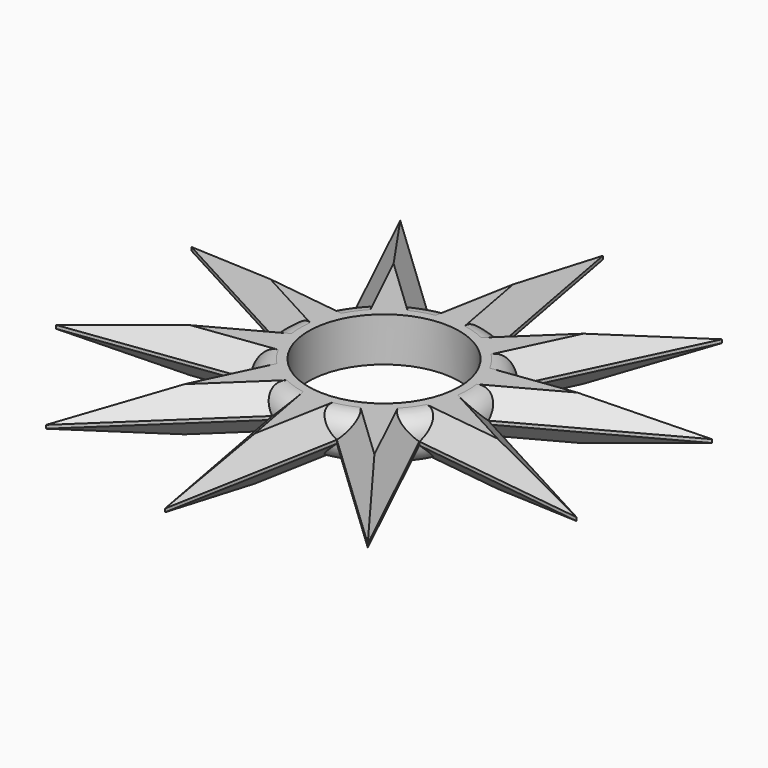
from build123d import *

# Parameters (mm, degrees)
F0_R     = 11.1
F1_DEPTH = 6.5
F2_SIZE  = 3
F3_R     = 2.99999


# Not quite as in the source:
# - a fillet or chamfer is up to 0.001 mm smaller than in the source, because OpenCascade refuses the exact size


with BuildPart() as f1:
    # F0 (on Top) → F1 (new body)
    with BuildSketch(Plane.XY):
        with BuildLine():
            Line((0, 40.2588956058), (-4.7404649607, 14.6152020464))
            ThreePointArc((-4.7404649607, 14.6152020464), (-4.7479748611, 14.612764065), (-4.7554835077, 14.6103222247))
            Line((-4.7554835077, 14.6103222247), (-23.6635851107, 32.5701307199))
            Line((-23.6635851107, 32.5701307199), (-12.4257169366, 9.0375714388))
            ThreePointArc((-12.4257169366, 9.0375714388), (-12.4303595641, 9.0311848617), (-12.4349989091, 9.0247958997))
            Line((-12.4349989091, 9.0247958997), (-38.2884850047, 12.440682917))
            Line((-38.2884850047, 12.440682917), (-15.3647673773, 0.0078957174))
            ThreePointArc((-15.3647673773, 0.0078957174), (-15.364769406, 0), (-15.3647673773, -0.0078957174))
            Line((-15.3647673773, -0.0078957174), (-38.2884850047, -12.440682917))
            Line((-38.2884850047, -12.440682917), (-12.4349989091, -9.0247958997))
            ThreePointArc((-12.4349989091, -9.0247958997), (-12.4303595641, -9.0311848617), (-12.4257169366, -9.0375714388))
            Line((-12.4257169366, -9.0375714388), (-23.6635851107, -32.5701307199))
            Line((-23.6635851107, -32.5701307199), (-4.7554835077, -14.6103222247))
            ThreePointArc((-4.7554835077, -14.6103222247), (-4.7479748611, -14.612764065), (-4.7404649607, -14.6152020464))
            Line((-4.7404649607, -14.6152020464), (0, -40.2588956058))
            Line((0, -40.2588956058), (4.7404649607, -14.6152020464))
            ThreePointArc((4.7404649607, -14.6152020464), (4.7479748611, -14.612764065), (4.7554835077, -14.6103222247))
            Line((4.7554835077, -14.6103222247), (23.6635851107, -32.5701307199))
            Line((23.6635851107, -32.5701307199), (12.4257169366, -9.0375714388))
            ThreePointArc((12.4257169366, -9.0375714388), (12.4303595641, -9.0311848617), (12.4349989091, -9.0247958997))
            Line((12.4349989091, -9.0247958997), (38.2884850047, -12.440682917))
            Line((38.2884850047, -12.440682917), (15.3647673773, -0.0078957174))
            ThreePointArc((15.3647673773, -0.0078957174), (15.364769406, 0), (15.3647673773, 0.0078957174))
            Line((15.3647673773, 0.0078957174), (38.2884850047, 12.440682917))
            Line((38.2884850047, 12.440682917), (12.4349989091, 9.0247958997))
            ThreePointArc((12.4349989091, 9.0247958997), (12.4303595641, 9.0311848617), (12.4257169366, 9.0375714388))
            Line((12.4257169366, 9.0375714388), (23.6635851107, 32.5701307199))
            Line((23.6635851107, 32.5701307199), (4.7554835077, 14.6103222247))
            ThreePointArc((4.7554835077, 14.6103222247), (4.7479748611, 14.612764065), (4.7404649607, 14.6152020464))
            Line((4.7404649607, 14.6152020464), (0, 40.2588956058))
        make_face()
        Circle(F0_R, mode=Mode.SUBTRACT)
    extrude(amount=F1_DEPTH)

    # F2
    f2_edges = [f1.edges().sort_by_distance(p)[0] for p in [
        (-26.826626, -6.224289, 6.5),
        (-26.826626, 6.224289, 6.5),
        (-25.361742, 10.732739, 6.5),
        (-18.044651, 20.803851, 6.5),
        (-14.209534, 23.590226, 6.5),
        (-2.370232, 27.437049, 6.5),
        (2.370232, 27.437049, 6.5),
        (14.209534, 23.590226, 6.5),
        (18.044651, 20.803851, 6.5),
        (25.361742, 10.732739, 6.5),
        (26.826626, 6.224289, 6.5),
        (26.826626, -6.224289, 6.5),
        (25.361742, -10.732739, 6.5),
        (18.044651, -20.803851, 6.5),
        (14.209534, -23.590226, 6.5),
        (2.370232, -27.437049, 6.5),
        (-18.044651, -20.803851, 6.5),
        (-26.826626, 6.224289, 0),
        (-25.361742, 10.732739, 0),
        (-26.826626, -6.224289, 0),
        (-25.361742, -10.732739, 0),
        (-14.209534, -23.590226, 0),
        (-18.044651, -20.803851, 0),
        (-2.370232, -27.437049, 0),
        (2.370232, -27.437049, 0),
        (14.209534, -23.590226, 0),
        (18.044651, -20.803851, 0),
        (25.361742, -10.732739, 0),
        (26.826626, -6.224289, 0),
        (26.826626, 6.224289, 0),
        (25.361742, 10.732739, 0),
        (18.044651, 20.803851, 0),
        (14.209534, 23.590226, 0),
        (2.370232, 27.437049, 0),
        (-2.370232, 27.437049, 0),
        (-14.209534, 23.590226, 0),
        (-18.044651, 20.803851, 0),
        (-25.361742, -10.732739, 6.5),
        (-14.209534, -23.590226, 6.5),
        (-2.370232, -27.437049, 6.5),
    ]]
    chamfer(f2_edges, length=F2_SIZE)

    # F3 (radius 3 in the source; OpenCascade refuses exactly that, so slightly less here)
    f3_edges = [f1.edges().sort_by_distance(p)[0] for p in [
        (-15.364769, 0, 0),
        (-12.43036, -9.031185, 0),
        (-4.747975, -14.612764, 0),
        (4.747975, -14.612764, 0),
        (12.43036, -9.031185, 0),
        (15.364769, 0, 0),
        (12.43036, 9.031185, 0),
        (4.747975, 14.612764, 0),
        (-4.747975, 14.612764, 0),
        (-12.43036, 9.031185, 0),
        (12.43036, 9.031185, 6.5),
        (4.747975, 14.612764, 6.5),
        (-4.747975, 14.612764, 6.5),
        (-12.43036, 9.031185, 6.5),
        (-15.364769, 0, 6.5),
        (-12.43036, -9.031185, 6.5),
        (-4.747975, -14.612764, 6.5),
        (4.747975, -14.612764, 6.5),
        (12.43036, -9.031185, 6.5),
        (15.364769, 0, 6.5),
    ]]
    fillet(f3_edges, radius=F3_R)


solid = f1.part
